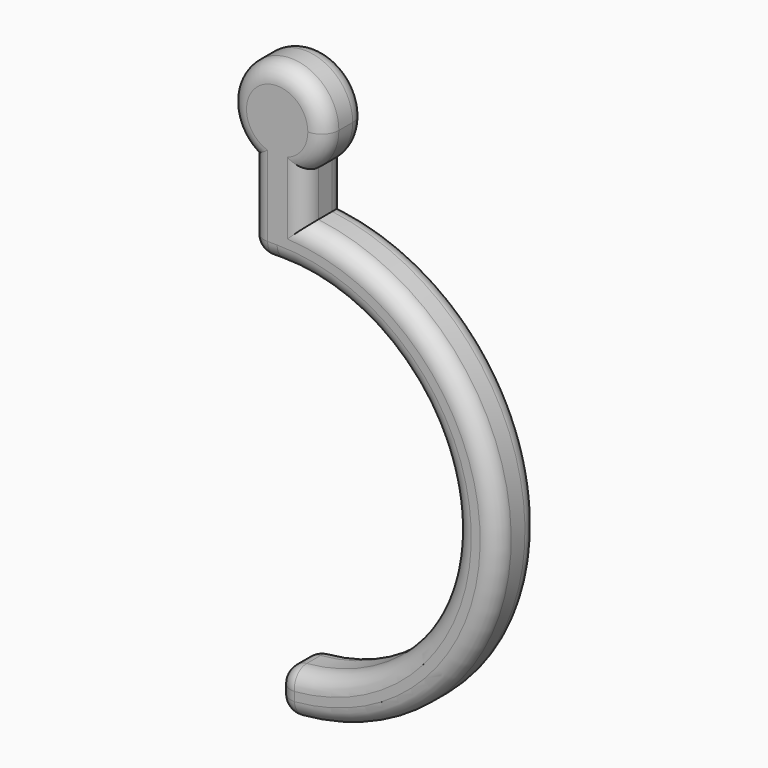
from build123d import *

# Parameters (mm, degrees)
F1_DEPTH      = 7.62
F1_DEPTH_BACK = 7.62
F2_R          = 5.08


with BuildPart() as f1:
    # F0 (on Front) → F1 (new body, two sides)
    with BuildSketch(Plane.XZ) as f1_sk:
        with BuildLine():
            Line((0, -52.113356), (0, -64.884435))
            ThreePointArc((0, -64.884435), (64.758143, -4.046326), (8.076901, 64.37976))
            Line((8.076901, 64.37976), (0, 64.37976))
            Line((0, 64.37976), (0, 52.113356))
            ThreePointArc((0, 52.113356), (52.113356, 0), (0, -52.113356))
        make_face()
        with BuildLine():
            Line((0, 64.37976), (8.076901, 64.37976))
            ThreePointArc((8.076901, 64.37976), (4.046326, 64.758143), (0, 64.884435))
            Line((0, 64.884435), (0, 64.37976))
        make_face()
        with BuildLine():
            ThreePointArc((0, 64.884435), (4.046326, 64.758143), (8.076901, 64.37976))
            Line((8.076901, 64.37976), (8.076901, 77.880624))
            ThreePointArc((8.076901, 77.880624), (4.233427, 75.990635), (0, 75.340682))
            Line((0, 75.340682), (0, 64.884435))
        make_face()
        Polygon((0, 64.37976), (0, 64.884435), (-7.90021, 64.884435), (-7.90021, 52.113356), (0, 52.113356), align=None)
        with BuildLine():
            Line((-7.90021, 64.884435), (0, 64.884435))
            Line((0, 64.884435), (0, 75.340682))
            ThreePointArc((0, 75.340682), (-4.13107, 75.958874), (-7.90021, 77.759286))
            Line((-7.90021, 77.759286), (-7.90021, 64.884435))
        make_face()
        with BuildLine():
            ThreePointArc((0, 75.340682), (4.233427, 75.990635), (8.076901, 77.880624))
            Line((8.076901, 77.880624), (8.076901, 89.452744))
            Line((8.076901, 89.452744), (0, 89.452744))
            Line((0, 89.452744), (0, 75.340682))
        make_face()
        with BuildLine():
            Line((8.076901, 89.452744), (8.076901, 77.880624))
            ThreePointArc((8.076901, 77.880624), (12.512633, 82.927081), (14.112061, 89.452744))
            ThreePointArc((14.112061, 89.452744), (-6.620499, 101.915458), (-7.90021, 77.759286))
            Line((-7.90021, 77.759286), (-7.90021, 89.452744))
            Line((-7.90021, 89.452744), (0, 89.452744))
            Line((0, 89.452744), (8.076901, 89.452744))
        make_face()
        with BuildLine():
            ThreePointArc((-7.90021, 77.759286), (-4.13107, 75.958874), (0, 75.340682))
            Line((0, 75.340682), (0, 89.452744))
            Line((0, 89.452744), (-7.90021, 89.452744))
            Line((-7.90021, 89.452744), (-7.90021, 77.759286))
        make_face()
    extrude(amount=F1_DEPTH)
    extrude(f1_sk.sketch, amount=-F1_DEPTH_BACK)

    # F2
    f2_edges = [f1.edges().sort_by_distance(p)[0] for p in [
        (64.758143, -7.62, -4.046326),
        (64.758143, 7.62, -4.046326),
        (8.076901, -7.62, 71.130192),
        (8.076901, 7.62, 71.130192),
        (-0.107171, -7.62, 103.564398),
        (-0.107171, 7.62, 103.564398),
        (-7.90021, -7.62, 64.936321),
        (52.113356, -7.62, 0),
        (-7.90021, 0, 52.113356),
        (-3.950105, 7.62, 52.113356),
        (52.113356, 7.62, 0),
        (-7.90021, 7.62, 64.936321),
        (0, 0, -64.884435),
        (0, 0, -52.113356),
        (0, -7.62, -58.498895),
        (0, 7.62, -58.498895),
        (-3.950105, -7.62, 52.113356),
    ]]
    fillet(f2_edges, radius=F2_R)


solid = f1.part
